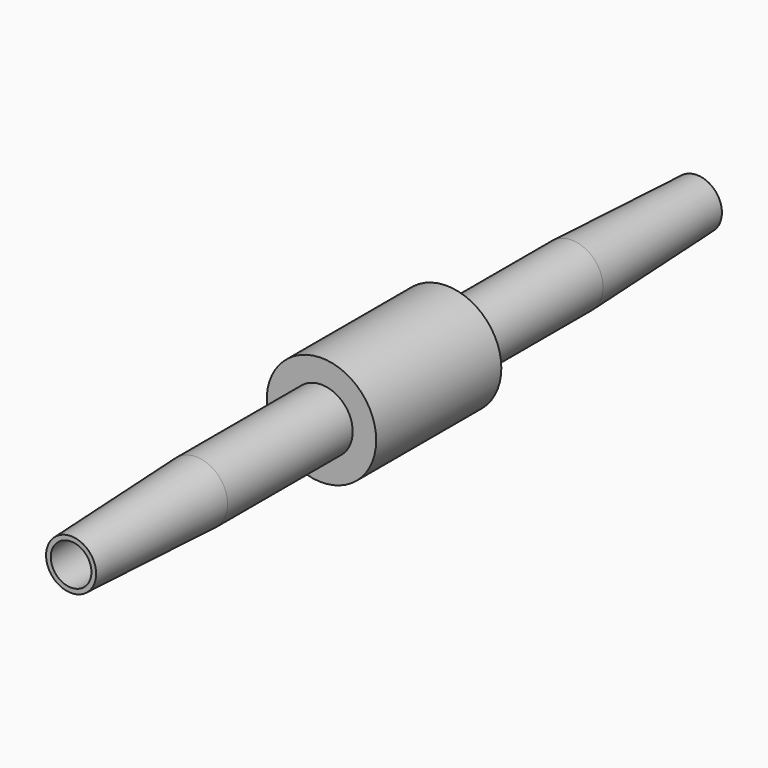
from build123d import *
from build123d import SkipClean  # not in build123d's __all__

# Parameters (mm, degrees)
F0_R     = 0.175
F0_R_2   = 0.1
F0_R_3   = 0.065
F1_DEPTH = 0.25
F2_DEPTH = 0.75


with BuildPart() as f1:
    # F0 (on Front) → F1 (new body, symmetric)
    with BuildSketch(Plane.XZ):
        Circle(F0_R)
        Circle(F0_R_2, mode=Mode.SUBTRACT)
        Circle(F0_R_2)
        Circle(F0_R_3, mode=Mode.SUBTRACT)
    extrude(amount=F1_DEPTH, both=True)

    # F0 (on Front) → F2 (join, symmetric)
    with BuildSketch(Plane.XZ):
        Circle(F0_R_2)
        Circle(F0_R_3, mode=Mode.SUBTRACT)
    extrude(amount=F2_DEPTH, both=True)

    # F3 (on Right) → F4 (revolve)
    with BuildSketch(Plane.YZ):
        Polygon((0.75, 0.065), (1.25, 0.065), (1.25, 0.08), (0.75, 0.1), align=None)
    with SkipClean():  # cleaning this boolean's faces spoils the solid; the shape is the same uncleaned
        revolve(axis=Axis((0, 0.625, 0), (0, 1, 0)))

    # F5: F1 across plane


with BuildPart() as f1_1:
    add(f1.part, clean=False)
    with SkipClean():  # cleaning this boolean's faces spoils the solid; the shape is the same uncleaned
        add(f1.part.mirror(Plane.XZ), clean=False)


solid = f1_1.part
